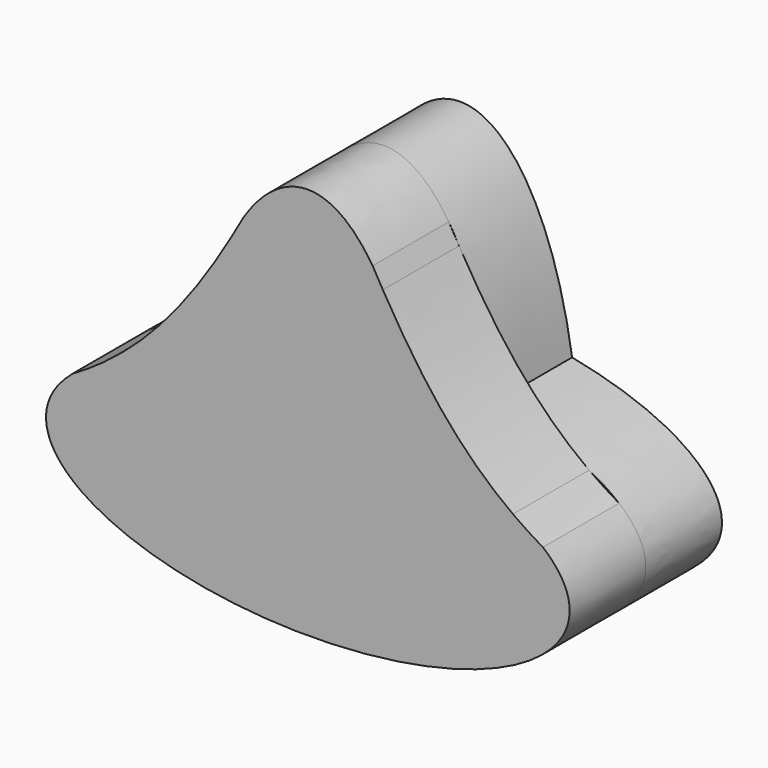
from build123d import *

# Parameters (mm, degrees)
F1_DEPTH = 50.8
F3_DEPTH = 50.8


with BuildPart() as f1:
    # F0 (on Front) → F1 (new body)
    with BuildSketch(Plane.XZ):
        with BuildLine():
            add(Edge.make_bspline(
                [(59.7403431378, 51.6608795344), (44.6162356791, 152.4), (0, 152.4)],
                knots=[5.0582237592, 5.0582237592, 5.0582237592, 6.2831853072, 6.2831853072, 6.2831853072], degree=2, weights=[1, 0.8182243425, 1]))
            add(Edge.make_bspline(
                [(0, 152.4), (-44.6162356791, 152.4), (-59.7403431378, 51.6608795344)],
                knots=[0, 0, 0, 1.224961548, 1.224961548, 1.224961548], degree=2, weights=[1, 0.8182243425, 1]))
            add(Edge.make_bspline(
                [(59.7403431378, 51.6608795344), (0, 63.2223556671), (-59.7403431378, 51.6608795344)],
                knots=[1.128923574, 1.128923574, 1.128923574, 2.0126690796, 2.0126690796, 2.0126690796], degree=2, weights=[1, 0.9039523978, 1]))
        make_face()
        with BuildLine():
            add(Edge.make_bspline(
                [(59.7403431378, 51.6608795344), (0, 63.2223556671), (-59.7403431378, 51.6608795344)],
                knots=[1.128923574, 1.128923574, 1.128923574, 2.0126690796, 2.0126690796, 2.0126690796], degree=2, weights=[1, 0.9039523978, 1]))
            add(Edge.make_bspline(
                [(-59.7403431378, 51.6608795344), (-67.4962644708, 0), (-59.7403431378, -51.6608795344)],
                knots=[1.224961548, 1.224961548, 1.224961548, 1.9166311056, 1.9166311056, 1.9166311056], degree=2, weights=[1, 0.9407928053, 1]))
            add(Edge.make_bspline(
                [(-59.7403431378, -51.6608795344), (0, -63.2223556671), (59.7403431378, -51.6608795344)],
                knots=[4.2705162276, 4.2705162276, 4.2705162276, 5.1542617331, 5.1542617331, 5.1542617331], degree=2, weights=[1, 0.9039523978, 1]))
            add(Edge.make_bspline(
                [(59.7403431378, -51.6608795344), (67.4962644708, 0), (59.7403431378, 51.6608795344)],
                knots=[4.3665542016, 4.3665542016, 4.3665542016, 5.0582237592, 5.0582237592, 5.0582237592], degree=2, weights=[1, 0.9407928053, 1]))
        make_face()
        with BuildLine():
            add(Edge.make_bspline(
                [(-59.7403431378, 51.6608795344), (-67.4962644708, 0), (-59.7403431378, -51.6608795344)],
                knots=[1.224961548, 1.224961548, 1.224961548, 1.9166311056, 1.9166311056, 1.9166311056], degree=2, weights=[1, 0.9407928053, 1]))
            add(Edge.make_bspline(
                [(-59.7403431378, 51.6608795344), (-326.6819200385, 0), (-59.7403431378, -51.6608795344)],
                knots=[2.0126690796, 2.0126690796, 2.0126690796, 4.2705162276, 4.2705162276, 4.2705162276], degree=2, weights=[1, 0.4276330933, 1]))
        make_face()
        with BuildLine():
            add(Edge.make_bspline(
                [(139.7, 0), (139.7, 36.1863841458), (59.7403431378, 51.6608795344)],
                knots=[0, 0, 0, 1.128923574, 1.128923574, 1.128923574], degree=2, weights=[1, 0.8448766458, 1]))
            add(Edge.make_bspline(
                [(59.7403431378, -51.6608795344), (67.4962644708, 0), (59.7403431378, 51.6608795344)],
                knots=[4.3665542016, 4.3665542016, 4.3665542016, 5.0582237592, 5.0582237592, 5.0582237592], degree=2, weights=[1, 0.9407928053, 1]))
            add(Edge.make_bspline(
                [(59.7403431378, -51.6608795344), (139.7, -36.1863841458), (139.7, 0)],
                knots=[5.1542617331, 5.1542617331, 5.1542617331, 6.2831853072, 6.2831853072, 6.2831853072], degree=2, weights=[1, 0.8448766458, 1]))
        make_face()
    extrude(amount=F1_DEPTH)

    # F2 (on face) → F3 (join)
    with BuildSketch(Plane.XZ.offset(50.8)):
        with BuildLine():
            add(Edge.make_bspline(
                [(-125.4921527709, 25.1110170179), (-119.8408847602, 28.3667906254), (-114.4923876387, 31.8490724953), (-109.4129774478, 35.5341797873)],
                knots=[0, 0, 0, 0, 18.1073300487, 18.1073300487, 18.1073300487, 18.1073300487], degree=3))
            add(Edge.make_bspline(
                [(-125.4921527709, 25.1110170179), (-146.2695882638, 7.7336542687), (-150.2952536866, -13.9005389833), (-127.7909797078, -33.3610054732), (-90.9168381727, -45.6273302724), (-38.1393725678, -55.8412891633), (-13.1441546468, -58.3577240351), (13.1441546468, -58.3577240351), (38.1393725678, -55.8412891633), (86.7627618143, -46.4312636305), (112.9741363986, -37.7048006914), (131.6263227318, -25.6538691464), (139.7, -12.2292123447), (139.7, 4.9682976791), (138.3781576401, 10.1092094273), (135.5600424417, 15.2807206428), (131.2097879034, 20.3403255939), (125.435047557, 25.1587212091)],
                knots=[2.7289069801, 2.7289069801, 2.7289069801, 2.7289069801, 2.7289069801, 2.7289069801, 4.2705162276, 4.2705162276, 4.2705162276, 4.2705162276, 5.3386368085, 5.3386368085, 5.3386368085, 5.3386368085, 6.6748360981, 6.6748360981, 6.6748360981, 6.6748360981, 7.2176867448, 7.2176867448, 7.2176867448, 7.2176867448, 7.2176867448, 7.2176867448], degree=5, weights=[0.9385256306, 0.9101891335, 0.9001522237, 0.93891022, 1, 1, 0.9963099432, 0.9963099432, 1, 1, 0.990374698, 0.990374698, 1, 1, 0.998411334, 0.9965248399, 0.9951069337, 0.9943996096]))
            add(Edge.make_bspline(
                [(109.4610297505, 35.5094042439), (114.5073930841, 31.8507982963), (119.8208768364, 28.3927656455), (125.435047557, 25.1587212091)],
                knots=[119.1216734954, 119.1216734954, 119.1216734954, 119.1216734954, 137.1016867436, 137.1016867436, 137.1016867436, 137.1016867436], degree=3))
            add(Edge.make_bspline(
                [(109.4610297505, 35.5094042439), (101.2636080171, 39.738359396), (91.9070529121, 43.5406099316), (81.6340028034, 46.8188914315), (70.7800298464, 49.5243823586), (59.7403431378, 51.6608795344)],
                knots=[7.4651471121, 7.4651471121, 7.4651471121, 7.4651471121, 7.4651471121, 7.4651471121, 8.0110353878, 8.0110353878, 8.0110353878, 8.0110353878, 8.0110353878, 8.0110353878], degree=5, weights=[0.9943800426, 0.9950752856, 0.9964931433, 0.9983935048, 1, 1]))
            add(Edge.make_bspline(
                [(59.7403431378, 51.6608795344), (57.5382578812, 66.3285967891), (54.4517732012, 80.9902621108), (50.4382644861, 94.9216248161), (45.572005147, 107.5005144347), (40.0358811137, 118.2929354064)],
                knots=[5.0582237592, 5.0582237592, 5.0582237592, 5.0582237592, 5.0582237592, 5.0582237592, 5.5800734332, 5.5800734332, 5.5800734332, 5.5800734332, 5.5800734332, 5.5800734332], degree=5, weights=[1, 1, 0.9973842549, 0.9944800917, 0.9925794821, 0.9919390426]))
            add(Edge.make_bspline(
                [(34.5744466343, 127.82918292), (36.3761042693, 124.632101445), (38.1941104643, 121.4516279127), (40.0358811137, 118.2929354064)],
                knots=[0, 0, 0, 0, 10.8694846013, 10.8694846013, 10.8694846013, 10.8694846013], degree=3))
            add(Edge.make_bspline(
                [(34.5744466343, 127.82918292), (28.2336843158, 137.7076414844), (21.3159684375, 145.2708413155), (14.0902928117, 150.1589141307), (6.8772995732, 152.4), (-6.7989683258, 152.4), (-13.9255548606, 150.2098204169), (-21.0683157096, 145.4373430481), (-27.917696592, 138.0507600382), (-34.2124461608, 128.3889758488)],
                knots=[5.6787987596, 5.6787987596, 5.6787987596, 5.6787987596, 5.6787987596, 5.6787987596, 6.2312653993, 6.2312653993, 6.2312653993, 6.2312653993, 6.77743954, 6.77743954, 6.77743954, 6.77743954, 6.77743954, 6.77743954], degree=5, weights=[0.9917950036, 0.9921552043, 0.9939664209, 0.9970683191, 1, 1, 0.9971347214, 0.9940723408, 0.992238718, 0.9918173966]))
            add(Edge.make_bspline(
                [(-40.4146945279, 117.548620602), (-38.3185692298, 121.1355421887), (-36.2547180821, 124.7515004342), (-34.2124461608, 128.3889758488)],
                knots=[125.4813945277, 125.4813945277, 125.4813945277, 125.4813945277, 137.834399259, 137.834399259, 137.834399259, 137.834399259], degree=3))
            add(Edge.make_bspline(
                [(-40.4146945279, 117.548620602), (-45.8386376728, 106.8072580552), (-50.6034245471, 94.3460949074), (-54.536523657, 80.5868796167), (-57.5684734099, 66.1273362655), (-59.7403431378, 51.6608795344)],
                knots=[6.8896178347, 6.8896178347, 6.8896178347, 6.8896178347, 6.8896178347, 6.8896178347, 7.4043070395, 7.4043070395, 7.4043070395, 7.4043070395, 7.4043070395, 7.4043070395], degree=5, weights=[0.9919853468, 0.992684918, 0.9945994697, 0.9974555454, 1, 1]))
            add(Edge.make_bspline(
                [(-59.7403431378, 51.6608795344), (-69.9985392989, 49.6756232761), (-80.5612184861, 47.1064874977), (-90.9490655448, 43.8933915356), (-100.7021400438, 40.022895552), (-109.4129774478, 35.5341797873)],
                knots=[2.0126690796, 2.0126690796, 2.0126690796, 2.0126690796, 2.0126690796, 2.0126690796, 2.5199143631, 2.5199143631, 2.5199143631, 2.5199143631, 2.5199143631, 2.5199143631], degree=5, weights=[1, 1, 0.993386125, 0.9831301058, 0.9715360475, 0.9602404299]))
        make_face()
        with BuildLine():
            add(Edge.make_bspline(
                [(109.4610297505, 35.5094042439), (101.2636080171, 39.738359396), (91.9070529121, 43.5406099316), (81.6340028034, 46.8188914315), (70.7800298464, 49.5243823586), (59.7403431378, 51.6608795344)],
                knots=[7.4651471121, 7.4651471121, 7.4651471121, 7.4651471121, 7.4651471121, 7.4651471121, 8.0110353878, 8.0110353878, 8.0110353878, 8.0110353878, 8.0110353878, 8.0110353878], degree=5, weights=[0.9943800426, 0.9950752856, 0.9964931433, 0.9983935048, 1, 1]))
            add(Edge.make_bspline(
                [(40.0358811137, 118.2929354064), (58.378581946, 86.834647328), (79.0784116022, 57.5367574312), (109.4610297505, 35.5094042439)],
                knots=[10.8694846013, 10.8694846013, 10.8694846013, 10.8694846013, 119.1216734954, 119.1216734954, 119.1216734954, 119.1216734954], degree=3))
            add(Edge.make_bspline(
                [(59.7403431378, 51.6608795344), (57.5382578812, 66.3285967891), (54.4517732012, 80.9902621108), (50.4382644861, 94.9216248161), (45.572005147, 107.5005144347), (40.0358811137, 118.2929354064)],
                knots=[5.0582237592, 5.0582237592, 5.0582237592, 5.0582237592, 5.0582237592, 5.0582237592, 5.5800734332, 5.5800734332, 5.5800734332, 5.5800734332, 5.5800734332, 5.5800734332], degree=5, weights=[1, 1, 0.9973842549, 0.9944800917, 0.9925794821, 0.9919390426]))
        make_face()
        with BuildLine():
            add(Edge.make_bspline(
                [(-109.4129774478, 35.5341797873), (-79.2927490157, 57.3863770424), (-58.6345121192, 86.3705907938), (-40.4146945279, 117.548620602)],
                knots=[18.1073300487, 18.1073300487, 18.1073300487, 18.1073300487, 125.4813945277, 125.4813945277, 125.4813945277, 125.4813945277], degree=3))
            add(Edge.make_bspline(
                [(-59.7403431378, 51.6608795344), (-69.9985392989, 49.6756232761), (-80.5612184861, 47.1064874977), (-90.9490655448, 43.8933915356), (-100.7021400438, 40.022895552), (-109.4129774478, 35.5341797873)],
                knots=[2.0126690796, 2.0126690796, 2.0126690796, 2.0126690796, 2.0126690796, 2.0126690796, 2.5199143631, 2.5199143631, 2.5199143631, 2.5199143631, 2.5199143631, 2.5199143631], degree=5, weights=[1, 1, 0.993386125, 0.9831301058, 0.9715360475, 0.9602404299]))
            add(Edge.make_bspline(
                [(-40.4146945279, 117.548620602), (-45.8386376728, 106.8072580552), (-50.6034245471, 94.3460949074), (-54.536523657, 80.5868796167), (-57.5684734099, 66.1273362655), (-59.7403431378, 51.6608795344)],
                knots=[6.8896178347, 6.8896178347, 6.8896178347, 6.8896178347, 6.8896178347, 6.8896178347, 7.4043070395, 7.4043070395, 7.4043070395, 7.4043070395, 7.4043070395, 7.4043070395], degree=5, weights=[0.9919853468, 0.992684918, 0.9945994697, 0.9974555454, 1, 1]))
        make_face()
    extrude(amount=F3_DEPTH)


solid = f1.part
